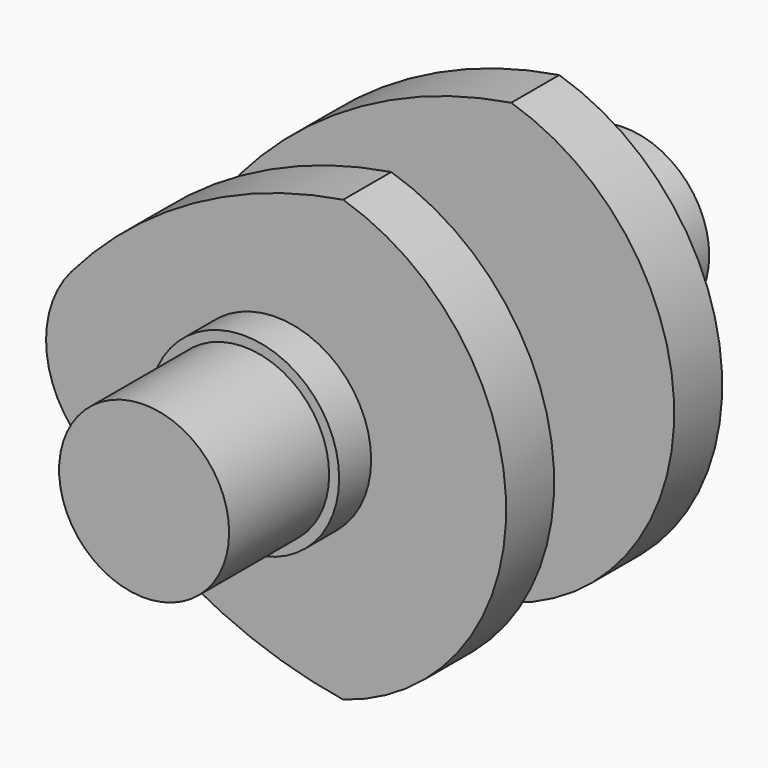
from build123d import *

# Parameters (mm, degrees)
F0_R     = 17
F1_DEPTH = 25
F2_R     = 19
F3_DEPTH = 8
F4_R     = 19
F5_DEPTH = 12
F6_R     = 16
F7_DEPTH = 15


with BuildPart() as f1:
    # F0 (on Front) → F1 (new body)
    with BuildSketch(Plane.XZ):
        Circle(F0_R)
    extrude(amount=F1_DEPTH)

    # F2 (on face) → F3 (join)
    with BuildSketch(Plane.XZ):
        Circle(F2_R)
    extrude(amount=-F3_DEPTH)

    # F4 (on face) → F5 (join)
    with BuildSketch(Plane(origin=(0, 8, 0), x_dir=(-1, 0, 0), z_dir=(0, 1, 0))):
        with BuildLine():
            ThreePointArc((40.9431234611, 13.6680947576), (16.4692576238, 33.6834442487), (-13.416407865, 44))
            ThreePointArc((-13.416407865, 44), (-46, 0), (-13.416407865, -44))
            ThreePointArc((-13.416407865, -44), (16.4692576238, -33.6834442487), (40.9431234611, -13.6680947576))
            ThreePointArc((40.9431234611, -13.6680947576), (46, 0), (40.9431234611, 13.6680947576))
        make_face()
        Circle(F4_R, mode=Mode.SUBTRACT)
        Circle(F4_R)
    extrude(amount=F5_DEPTH)

    # F6 (on face) → F7 (join)
    with BuildSketch(Plane(origin=(0, 20, 0), x_dir=(-1, 0, 0), z_dir=(0, 1, 0))):
        with Locations((25, 0)):
            Circle(F6_R)
    extrude(amount=F7_DEPTH)

    # F8: F1 across face


with BuildPart() as f1_1:
    add(f1.part)
    add(f1.part.mirror(Plane(origin=(-25, 35, 0), x_dir=(-1, 0, 0), z_dir=(0, 1, 0))))


solid = f1_1.part
